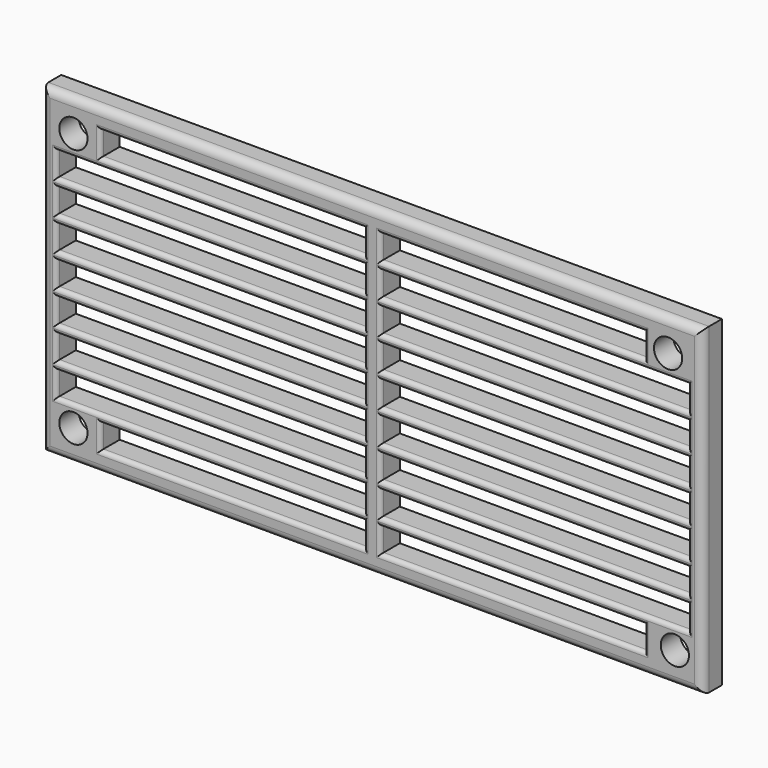
from build123d import *

# Parameters (mm, degrees)
F0_W     = 82
F0_H     = 40
F0_R     = 1.75
F0_W_2   = 2.0507176579
F0_H_2   = 3
F0_H_3   = 1
F1_DEPTH = 3
F2_R     = 0.49999
F3_R     = 1


# Not quite as in the source:
# - a fillet or chamfer is up to 0.001 mm smaller than in the source, because OpenCascade refuses the exact size


with BuildPart() as f1:
    # F0 (on Front) → F1 (new body)
    with BuildSketch(Plane.XZ):
        with Locations((-54.7693173022, 38.4868923018)):
            Rectangle(F0_W, F0_H)
        with Locations((-91.8560757875, 22.4002130298)):
            Circle(F0_R, mode=Mode.SUBTRACT)
        with Locations((-17.2127172435, 22.4002130298)):
            Circle(F0_R, mode=Mode.SUBTRACT)
        with Locations((-91.8560757875, 54.5735715738)):
            Circle(F0_R, mode=Mode.SUBTRACT)
        Polygon((-53.7439584732, 39.9868923018), (-15.5743994219, 39.9868923018), (-15.5743994219, 36.9868923018), (-53.7439584732, 36.9868923018), (-53.7439584732, 35.9868923018), (-15.5743994219, 35.9868923018), (-15.5743994219, 32.9868923018), (-53.7439584732, 32.9868923018), (-53.7439584732, 31.9868923018), (-15.5743994219, 31.9868923018), (-15.5743994219, 28.9868923018), (-53.7439584732, 28.9868923018), (-53.7439584732, 27.9868923018), (-15.5743994219, 27.9868923018), (-15.5743994219, 24.9868923018), (-53.7439584732, 24.9868923018), (-53.7439584732, 23.9868923018), (-21.0193173022, 23.9868923018), (-21.0193173022, 20.9868923018), (-53.7439584732, 20.9868923018), (-55.7946761312, 20.9868923018), (-88.5193173022, 20.9868923018), (-88.5193173022, 23.9868923018), (-55.7946761312, 23.9868923018), (-55.7946761312, 24.9868923018), (-93.9642351825, 24.9868923018), (-93.9642351825, 27.9868923018), (-55.7946761312, 27.9868923018), (-55.7946761312, 28.9868923018), (-93.9642351825, 28.9868923018), (-93.9642351825, 31.9868923018), (-55.7946761312, 31.9868923018), (-55.7946761312, 32.9868923018), (-93.9642351825, 32.9868923018), (-93.9642351825, 35.9868923018), (-55.7946761312, 35.9868923018), (-55.7946761312, 36.9868923018), (-93.9642351825, 36.9868923018), (-93.9642351825, 39.9868923018), (-55.7946761312, 39.9868923018), (-55.7946761312, 40.9868923018), (-93.9642351825, 40.9868923018), (-93.9642351825, 43.9868923018), (-55.7946761312, 43.9868923018), (-55.7946761312, 44.9868923018), (-93.9642351825, 44.9868923018), (-93.9642351825, 47.9868923018), (-55.7946761312, 47.9868923018), (-55.7946761312, 48.9868923018), (-93.9642351825, 48.9868923018), (-93.9642351825, 51.9868923018), (-55.7946761312, 51.9868923018), (-55.7946761312, 52.9868923018), (-88.5193173022, 52.9868923018), (-88.5193173022, 55.9868923018), (-55.7946761312, 55.9868923018), (-53.7439584732, 55.9868923018), (-21.0193173022, 55.9868923018), (-21.0193173022, 52.9868923018), (-53.7439584732, 52.9868923018), (-53.7439584732, 51.9868923018), (-15.5743994219, 51.9868923018), (-15.5743994219, 48.9868923018), (-53.7439584732, 48.9868923018), (-53.7439584732, 47.9868923018), (-15.5743994219, 47.9868923018), (-15.5743994219, 44.9868923018), (-53.7439584732, 44.9868923018), (-53.7439584732, 43.9868923018), (-15.5743994219, 43.9868923018), (-15.5743994219, 40.9868923018), (-53.7439584732, 40.9868923018), align=None, mode=Mode.SUBTRACT)
        with Locations((-18.0520743152, 54.5735715738)):
            Circle(F0_R, mode=Mode.SUBTRACT)
        with Locations((-54.7693173022, 54.4868923018)):
            Rectangle(F0_W_2, F0_H_2)
        with Locations((-54.7693173022, 52.4868923018)):
            Rectangle(F0_W_2, F0_H_3)
        with Locations((-54.7693173022, 50.4868923018)):
            Rectangle(F0_W_2, F0_H_2)
        with Locations((-54.7693173022, 48.4868923018)):
            Rectangle(F0_W_2, F0_H_3)
        with Locations((-54.7693173022, 46.4868923018)):
            Rectangle(F0_W_2, F0_H_2)
        with Locations((-54.7693173022, 44.4868923018)):
            Rectangle(F0_W_2, F0_H_3)
        with Locations((-54.7693173022, 42.4868923018)):
            Rectangle(F0_W_2, F0_H_2)
        with Locations((-54.7693173022, 40.4868923018)):
            Rectangle(F0_W_2, F0_H_3)
        with Locations((-54.7693173022, 38.4868923018)):
            Rectangle(F0_W_2, F0_H_2)
        with Locations((-54.7693173022, 36.4868923018)):
            Rectangle(F0_W_2, F0_H_3)
        with Locations((-54.7693173022, 34.4868923018)):
            Rectangle(F0_W_2, F0_H_2)
        with Locations((-54.7693173022, 32.4868923018)):
            Rectangle(F0_W_2, F0_H_3)
        with Locations((-54.7693173022, 30.4868923018)):
            Rectangle(F0_W_2, F0_H_2)
        with Locations((-54.7693173022, 28.4868923018)):
            Rectangle(F0_W_2, F0_H_3)
        with Locations((-54.7693173022, 26.4868923018)):
            Rectangle(F0_W_2, F0_H_2)
        with Locations((-54.7693173022, 24.4868923018)):
            Rectangle(F0_W_2, F0_H_3)
        with Locations((-54.7693173022, 22.4868923018)):
            Rectangle(F0_W_2, F0_H_2)
    extrude(amount=F1_DEPTH)

    # F2 (radius 0.5 in the source; OpenCascade refuses exactly that, so slightly less here)
    f2_edges = [f1.edges().sort_by_distance(p)[0] for p in [
        (-72.156997, -3, 20.986892),
        (-72.156997, -3, 23.986892),
        (-74.879456, -3, 24.986892),
        (-74.879456, -3, 27.986892),
        (-74.879456, -3, 28.986892),
        (-74.879456, -3, 31.986892),
        (-74.879456, -3, 32.986892),
        (-74.879456, -3, 35.986892),
        (-74.879456, -3, 36.986892),
        (-37.381638, -3, 20.986892),
        (-37.381638, -3, 23.986892),
        (-34.659179, -3, 24.986892),
        (-34.659179, -3, 27.986892),
        (-34.659179, -3, 28.986892),
        (-34.659179, -3, 31.986892),
        (-34.659179, -3, 32.986892),
        (-34.659179, -3, 35.986892),
        (-34.659179, -3, 36.986892),
        (-74.879456, -3, 39.986892),
        (-74.879456, -3, 40.986892),
        (-74.879456, -3, 43.986892),
        (-74.879456, -3, 44.986892),
        (-74.879456, -3, 47.986892),
        (-74.879456, -3, 48.986892),
        (-74.879456, -3, 51.986892),
        (-72.156997, -3, 52.986892),
        (-93.964235, -3, 26.486892),
        (-93.964235, -3, 30.486892),
        (-93.964235, -3, 34.486892),
        (-88.519317, -3, 22.486892),
        (-55.794676, -3, 22.486892),
        (-55.794676, -3, 26.486892),
        (-55.794676, -3, 30.486892),
        (-55.794676, -3, 34.486892),
        (-55.794676, -3, 38.486892),
        (-55.794676, -3, 42.486892),
        (-55.794676, -3, 46.486892),
        (-55.794676, -3, 50.486892),
        (-55.794676, -3, 54.486892),
        (-72.156997, -3, 55.986892),
        (-53.743958, -3, 22.486892),
        (-53.743958, -3, 26.486892),
        (-53.743958, -3, 30.486892),
        (-53.743958, -3, 34.486892),
        (-53.743958, -3, 38.486892),
        (-34.659179, -3, 39.986892),
        (-34.659179, -3, 40.986892),
        (-53.743958, -3, 42.486892),
        (-34.659179, -3, 43.986892),
        (-34.659179, -3, 44.986892),
        (-53.743958, -3, 46.486892),
        (-34.659179, -3, 48.986892),
        (-34.659179, -3, 47.986892),
        (-53.743958, -3, 50.486892),
        (-34.659179, -3, 51.986892),
        (-37.381638, -3, 52.986892),
        (-53.743958, -3, 54.486892),
        (-37.381638, -3, 55.986892),
        (-93.964235, -3, 38.486892),
        (-93.964235, -3, 42.486892),
        (-93.964235, -3, 46.486892),
        (-93.964235, -3, 50.486892),
        (-88.519317, -3, 54.486892),
        (-21.019317, -3, 22.486892),
        (-15.574399, -3, 26.486892),
        (-15.574399, -3, 30.486892),
        (-15.574399, -3, 34.486892),
        (-15.574399, -3, 38.486892),
        (-15.574399, -3, 42.486892),
        (-15.574399, -3, 46.486892),
        (-15.574399, -3, 50.486892),
        (-21.019317, -3, 54.486892),
    ]]
    fillet(f2_edges, radius=F2_R)

    # F3
    f3_edges = [f1.edges().sort_by_distance(p)[0] for p in [
        (-54.769317, -3, 58.486892),
        (-13.769317, -3, 38.486892),
        (-54.769317, -3, 18.486892),
        (-95.769317, -3, 38.486892),
    ]]
    fillet(f3_edges, radius=F3_R)


solid = f1.part
